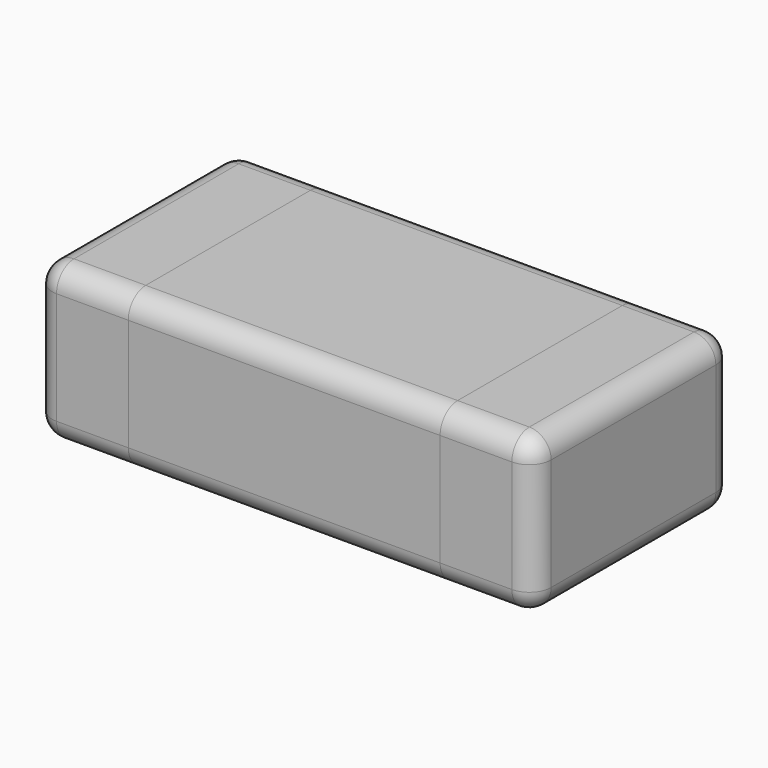
from build123d import *

# Parameters (mm, degrees)
F0_W           = 0.3
F0_H           = 0.8
F1_DEPTH       = 0.5
F0_W_2         = 1
F2_DEPTH       = 0.5
F3_R           = 0.07
F3_2_R         = 0.07
F4_T1_DEPTH    = 0.405
F4_S5_W        = 0.07
F4_S5_H        = 0.07
F4_T6_DEPTH    = 0.07
F4_S11_W       = 0.07
F4_S11_H       = 0.07
F4_T12_DEPTH   = 0.07
F4_S17_W       = 0.07
F4_S17_H       = 0.07
F4_T18_DEPTH   = 0.07
F4_S23_W       = 0.07
F4_S23_H       = 0.07
F4_T24_DEPTH   = 0.07
F4_2_F1_R      = 0.07
F4_2_F2_R      = 0.07
F4_2_F3_R      = 0.07
F4_2_F4_R      = 0.07
F4_3_T1_DEPTH  = 0.405
F4_3_S5_W      = 0.07
F4_3_S5_H      = 0.07
F4_3_T6_DEPTH  = 0.07
F4_3_S11_W     = 0.07
F4_3_S11_H     = 0.07
F4_3_T12_DEPTH = 0.07
F4_3_S17_W     = 0.07
F4_3_S17_H     = 0.07
F4_3_T18_DEPTH = 0.07
F4_3_S23_W     = 0.07
F4_3_S23_H     = 0.07
F4_3_T24_DEPTH = 0.07


# Not quite as in the source:
# - a fillet or chamfer that OpenCascade refuses, or shapes differently, is made with other operations: its cross-section is extruded or revolved along the edge and cut away or added


with BuildPart() as f1:
    # F0 (on Top) → F1 (new body)
    with BuildSketch(Plane.XY):
        with Locations((-0.65, 0)):
            Rectangle(F0_W, F0_H)
    extrude(amount=F1_DEPTH)

    # F3#2
    f3_2_edges = [f1.edges().sort_by_distance(p)[0] for p in [
        (-0.8, 0.4, 0.25),
        (-0.8, -0.4, 0.25),
        (-0.8, 0, 0),
        (-0.8, 0, 0.5),
    ]]
    fillet(f3_2_edges, radius=F3_2_R)

    # F4#3: fillet of radius 0.07 on 4 edges, made by hand

    # F4_3_s2 → F4_3_t1 (cut)
    with BuildSketch(Plane.YZ.offset(-0.73)):
        with BuildLine():
            ThreePointArc((0.33, 0.5), (0.3794974747, 0.4794974747), (0.4, 0.43))
            Line((0.4, 0.43), (0.4, 0.5))
            Line((0.4, 0.5), (0.33, 0.5))
        make_face()
        with BuildLine():
            ThreePointArc((0.33, 0), (0.3794974747, 0.0205025253), (0.4, 0.07))
            Line((0.4, 0.07), (0.4, 0))
            Line((0.4, 0), (0.33, 0))
        make_face()
        with BuildLine():
            ThreePointArc((-0.4, 0.43), (-0.3794974747, 0.4794974747), (-0.33, 0.5))
            Line((-0.33, 0.5), (-0.4, 0.5))
            Line((-0.4, 0.5), (-0.4, 0.43))
        make_face()
        with BuildLine():
            ThreePointArc((-0.4, 0.07), (-0.3794974747, 0.0205025253), (-0.33, 0))
            Line((-0.33, 0), (-0.4, 0))
            Line((-0.4, 0), (-0.4, 0.07))
        make_face()
    extrude(amount=F4_3_T1_DEPTH, mode=Mode.SUBTRACT)


with BuildPart() as f1b:
    # F0 (on Top) → F1, piece 2 (new body)
    with BuildSketch(Plane.XY):
        with Locations((0.65, 0)):
            Rectangle(F0_W, F0_H)
    extrude(amount=F1_DEPTH)

    # F3
    f3_edges = [f1b.edges().sort_by_distance(p)[0] for p in [
        (0.8, -0.4, 0.25),
        (0.8, 0.4, 0.25),
        (0.8, 0, 0),
        (0.8, 0, 0.5),
    ]]
    fillet(f3_edges, radius=F3_R)

    # F4: fillet of radius 0.07 on 4 edges, made by hand

    # F4_s2 → F4_t1 (cut)
    with BuildSketch(Plane.YZ.offset(0.325)):
        with BuildLine():
            ThreePointArc((0.33, 0.5), (0.3794974747, 0.4794974747), (0.4, 0.43))
            Line((0.4, 0.43), (0.4, 0.5))
            Line((0.4, 0.5), (0.33, 0.5))
        make_face()
        with BuildLine():
            ThreePointArc((0.33, 0), (0.3794974747, 0.0205025253), (0.4, 0.07))
            Line((0.4, 0.07), (0.4, 0))
            Line((0.4, 0), (0.33, 0))
        make_face()
        with BuildLine():
            ThreePointArc((-0.4, 0.43), (-0.3794974747, 0.4794974747), (-0.33, 0.5))
            Line((-0.33, 0.5), (-0.4, 0.5))
            Line((-0.4, 0.5), (-0.4, 0.43))
        make_face()
        with BuildLine():
            ThreePointArc((-0.4, 0.07), (-0.3794974747, 0.0205025253), (-0.33, 0))
            Line((-0.33, 0), (-0.4, 0))
            Line((-0.4, 0), (-0.4, 0.07))
        make_face()
    extrude(amount=F4_T1_DEPTH, mode=Mode.SUBTRACT)


with BuildPart() as f2:
    # F0 (on Top) → F2 (new body)
    with BuildSketch(Plane.XY):
        Rectangle(F0_W_2, F0_H)
    extrude(amount=F2_DEPTH)

    # F4#2: fillet of radius 0.07 on 4 edges, made by hand

    # F4_2_f1
    f4_2_f1_edges = [f2.edges().sort_by_distance(p)[0] for p in [
        (0, -0.4, 0),
    ]]
    fillet(f4_2_f1_edges, radius=F4_2_F1_R)

    # F4_2_f2
    f4_2_f2_edges = [f2.edges().sort_by_distance(p)[0] for p in [
        (0, -0.4, 0.5),
    ]]
    fillet(f4_2_f2_edges, radius=F4_2_F2_R)

    # F4_2_f3
    f4_2_f3_edges = [f2.edges().sort_by_distance(p)[0] for p in [
        (0, 0.4, 0),
    ]]
    fillet(f4_2_f3_edges, radius=F4_2_F3_R)

    # F4_2_f4
    f4_2_f4_edges = [f2.edges().sort_by_distance(p)[0] for p in [
        (0, 0.4, 0.5),
    ]]
    fillet(f4_2_f4_edges, radius=F4_2_F4_R)


with BuildPart() as f4_tool4:
    # F4_s5 → F4_t6 (new body)
    with BuildSketch(Plane.XZ.offset(0.33)):
        with Locations((0.765, 0.035)):
            Rectangle(F4_S5_W, F4_S5_H)
    extrude(amount=F4_T6_DEPTH)

    # F4_s7 → F4_t8 (revolve, cut)
    with BuildSketch(Plane(origin=(0.73, -0.33, 0.07), x_dir=(-0.7071067812, 0, 0.7071067812), z_dir=(0.7071067812, 0, 0.7071067812))):
        with BuildLine():
            ThreePointArc((0, -0.07), (0.07, 0), (0, 0.07))
            Line((0, 0.07), (0, -0.07))
        make_face()
    revolve(axis=Axis((0.73, -0.33, 0.07), (0, -1, 0)), mode=Mode.SUBTRACT)


with BuildPart() as f1b_1:
    add(f1b.part)

    # F4_t3: cut F4_tool4
    add(f4_tool4.part, mode=Mode.SUBTRACT)


with BuildPart() as f4_tool10:
    # F4_s11 → F4_t12 (new body)
    with BuildSketch(Plane.XZ.offset(0.33)):
        with Locations((0.765, 0.465)):
            Rectangle(F4_S11_W, F4_S11_H)
    extrude(amount=F4_T12_DEPTH)

    # F4_s13 → F4_t14 (revolve, cut)
    with BuildSketch(Plane(origin=(0.73, -0.33, 0.43), x_dir=(-0.7071067812, 0, -0.7071067812), z_dir=(-0.7071067812, 0, 0.7071067812))):
        with BuildLine():
            ThreePointArc((0, -0.07), (0.07, 0), (0, 0.07))
            Line((0, 0.07), (0, -0.07))
        make_face()
    revolve(axis=Axis((0.73, -0.33, 0.43), (0, -1, 0)), mode=Mode.SUBTRACT)


with BuildPart() as f1b_2:
    add(f1b_1.part)

    # F4_t9: cut F4_tool10
    add(f4_tool10.part, mode=Mode.SUBTRACT)


with BuildPart() as f4_tool16:
    # F4_s17 → F4_t18 (new body)
    with BuildSketch(Plane.XY.offset(0.07)):
        with Locations((0.765, 0.365)):
            Rectangle(F4_S17_W, F4_S17_H)
    extrude(amount=-F4_T18_DEPTH)

    # F4_s19 → F4_t20 (revolve, cut)
    with BuildSketch(Plane(origin=(0.73, 0.33, 0.07), x_dir=(-0.7071067812, -0.7071067812, 0), z_dir=(0.7071067812, -0.7071067812, 0))):
        with BuildLine():
            ThreePointArc((0, -0.07), (0.07, 0), (0, 0.07))
            Line((0, 0.07), (0, -0.07))
        make_face()
    revolve(axis=Axis((0.73, 0.33, 0.07), (0, 0, -1)), mode=Mode.SUBTRACT)


with BuildPart() as f1b_3:
    add(f1b_2.part)

    # F4_t15: cut F4_tool16
    add(f4_tool16.part, mode=Mode.SUBTRACT)


with BuildPart() as f4_tool22:
    # F4_s23 → F4_t24 (new body)
    with BuildSketch(Plane.XY.offset(0.43)):
        with Locations((0.765, 0.365)):
            Rectangle(F4_S23_W, F4_S23_H)
    extrude(amount=F4_T24_DEPTH)

    # F4_s25 → F4_t26 (revolve, cut)
    with BuildSketch(Plane(origin=(0.73, 0.33, 0.43), x_dir=(-0.7071067812, -0.7071067812, 0), z_dir=(-0.7071067812, 0.7071067812, 0))):
        with BuildLine():
            ThreePointArc((0, -0.07), (0.07, 0), (0, 0.07))
            Line((0, 0.07), (0, -0.07))
        make_face()
    revolve(axis=Axis((0.73, 0.33, 0.43), (0, 0, 1)), mode=Mode.SUBTRACT)


with BuildPart() as f1b_4:
    add(f1b_3.part)

    # F4_t21: cut F4_tool22
    add(f4_tool22.part, mode=Mode.SUBTRACT)


with BuildPart() as f4_3_tool4:
    # F4_3_s5 → F4_3_t6 (new body)
    with BuildSketch(Plane.XZ.offset(0.33)):
        with Locations((-0.765, 0.035)):
            Rectangle(F4_3_S5_W, F4_3_S5_H)
    extrude(amount=F4_3_T6_DEPTH)

    # F4_3_s7 → F4_3_t8 (revolve, cut)
    with BuildSketch(Plane(origin=(-0.73, -0.33, 0.07), x_dir=(0.7071067812, 0, 0.7071067812), z_dir=(0.7071067812, 0, -0.7071067812))):
        with BuildLine():
            ThreePointArc((0, -0.07), (0.07, 0), (0, 0.07))
            Line((0, 0.07), (0, -0.07))
        make_face()
    revolve(axis=Axis((-0.73, -0.33, 0.07), (0, -1, 0)), mode=Mode.SUBTRACT)


with BuildPart() as f1_1:
    add(f1.part)

    # F4_3_t3: cut F4_3_tool4
    add(f4_3_tool4.part, mode=Mode.SUBTRACT)


with BuildPart() as f4_3_tool10:
    # F4_3_s11 → F4_3_t12 (new body)
    with BuildSketch(Plane.XZ.offset(0.33)):
        with Locations((-0.765, 0.465)):
            Rectangle(F4_3_S11_W, F4_3_S11_H)
    extrude(amount=F4_3_T12_DEPTH)

    # F4_3_s13 → F4_3_t14 (revolve, cut)
    with BuildSketch(Plane(origin=(-0.73, -0.33, 0.43), x_dir=(0.7071067812, 0, -0.7071067812), z_dir=(-0.7071067812, 0, -0.7071067812))):
        with BuildLine():
            ThreePointArc((0, -0.07), (0.07, 0), (0, 0.07))
            Line((0, 0.07), (0, -0.07))
        make_face()
    revolve(axis=Axis((-0.73, -0.33, 0.43), (0, -1, 0)), mode=Mode.SUBTRACT)


with BuildPart() as f1_2:
    add(f1_1.part)

    # F4_3_t9: cut F4_3_tool10
    add(f4_3_tool10.part, mode=Mode.SUBTRACT)


with BuildPart() as f4_3_tool16:
    # F4_3_s17 → F4_3_t18 (new body)
    with BuildSketch(Plane.XY.offset(0.07)):
        with Locations((-0.765, 0.365)):
            Rectangle(F4_3_S17_W, F4_3_S17_H)
    extrude(amount=-F4_3_T18_DEPTH)

    # F4_3_s19 → F4_3_t20 (revolve, cut)
    with BuildSketch(Plane(origin=(-0.73, 0.33, 0.07), x_dir=(0.7071067812, -0.7071067812, 0), z_dir=(0.7071067812, 0.7071067812, 0))):
        with BuildLine():
            ThreePointArc((0, -0.07), (0.07, 0), (0, 0.07))
            Line((0, 0.07), (0, -0.07))
        make_face()
    revolve(axis=Axis((-0.73, 0.33, 0.07), (0, 0, -1)), mode=Mode.SUBTRACT)


with BuildPart() as f1_3:
    add(f1_2.part)

    # F4_3_t15: cut F4_3_tool16
    add(f4_3_tool16.part, mode=Mode.SUBTRACT)


with BuildPart() as f4_3_tool22:
    # F4_3_s23 → F4_3_t24 (new body)
    with BuildSketch(Plane.XY.offset(0.43)):
        with Locations((-0.765, 0.365)):
            Rectangle(F4_3_S23_W, F4_3_S23_H)
    extrude(amount=F4_3_T24_DEPTH)

    # F4_3_s25 → F4_3_t26 (revolve, cut)
    with BuildSketch(Plane(origin=(-0.73, 0.33, 0.43), x_dir=(0.7071067812, -0.7071067812, 0), z_dir=(-0.7071067812, -0.7071067812, 0))):
        with BuildLine():
            ThreePointArc((0, -0.07), (0.07, 0), (0, 0.07))
            Line((0, 0.07), (0, -0.07))
        make_face()
    revolve(axis=Axis((-0.73, 0.33, 0.43), (0, 0, 1)), mode=Mode.SUBTRACT)


with BuildPart() as f1_4:
    add(f1_3.part)

    # F4_3_t21: cut F4_3_tool22
    add(f4_3_tool22.part, mode=Mode.SUBTRACT)


solid = Compound([f2.part, f1b_4.part, f1_4.part])
